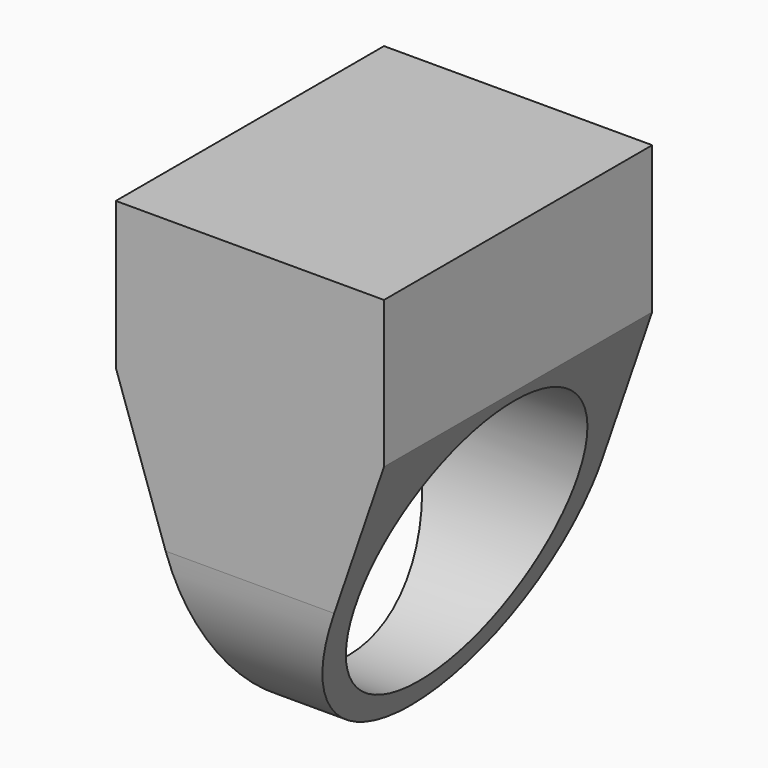
from build123d import *

# Parameters (mm, degrees)
F0_W        = 75
F0_H        = 30
F0_H_2      = 72.8525593877
F0_R        = 31.05
F1_DEPTH    = 30
F2_T1_DEPTH = 438.2716205132
F3_R        = 37.49999


# Not quite as in the source:
# - a fillet or chamfer that OpenCascade refuses, or shapes differently, is made with other operations: its cross-section is extruded or revolved along the edge and cut away or added
# - a fillet or chamfer is up to 0.001 mm smaller than in the source, because OpenCascade refuses the exact size


with BuildPart() as f1:
    # F0 (on Right) → F1 (new body, symmetric)
    with BuildSketch(Plane.YZ):
        with Locations((0, 51.4262796938)):
            Rectangle(F0_W, F0_H)
        Rectangle(F0_W, F0_H_2)
        Circle(F0_R, mode=Mode.SUBTRACT)
    extrude(amount=F1_DEPTH, both=True)

    # F2: chamfer of 70 x 24 on 2 edges, made by hand

    # F2_s2 → F2_t1 (cut)
    with BuildSketch(Plane.XZ.offset(-219.1358102566)):
        Polygon((30, 33.5737203062), (6, -36.4262796938), (30, -36.4262796938), align=None)
        Polygon((-6, -36.4262796938), (-30, 33.5737203062), (-30, -36.4262796938), align=None)
    extrude(amount=F2_T1_DEPTH, mode=Mode.SUBTRACT)

    # F3 (radius 37.5 in the source; OpenCascade refuses exactly that, so slightly less here)
    f3_edges = [f1.edges().sort_by_distance(p)[0] for p in [
        (0, -37.5, -36.42628),
        (0, 37.5, -36.42628),
    ]]
    fillet(f3_edges, radius=F3_R)


solid = f1.part
